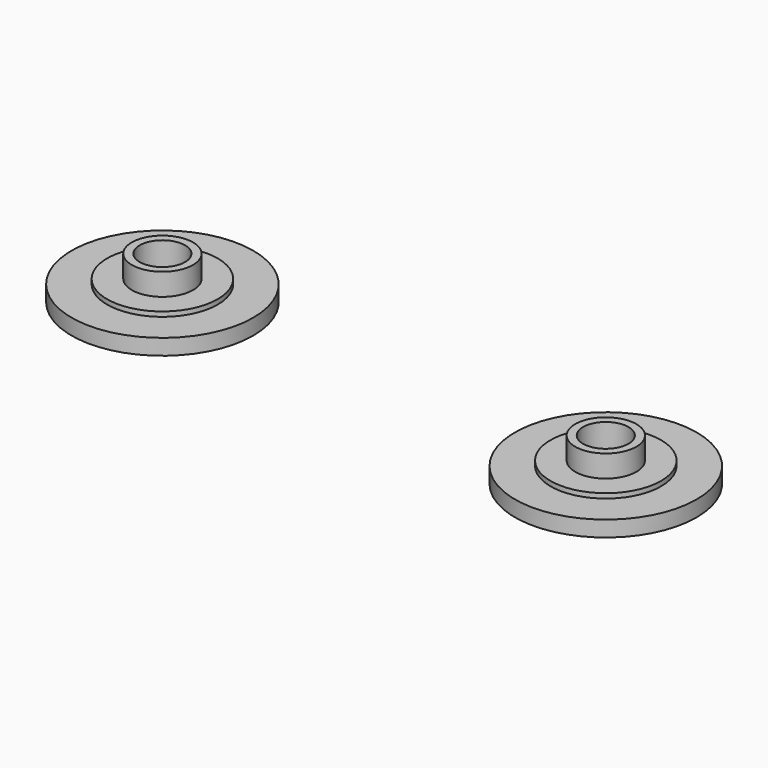
from build123d import *

# Parameters (mm, degrees)
F0_R        = 3.875
F1_DEPTH    = 3.4
F0_R_2      = 7
F2_DEPTH    = 0.6
F0_R_3      = 11.5
F3_DEPTH    = 2
F4_T        = 1
F5_R        = 3.875
F6_DEPTH    = 3.4
F5_R_2      = 7
F7_DEPTH    = 0.6
F6_FACE_R   = 3.875
F7_FACE_R   = 7
F7_FACE_R_2 = 3.875
F5_R_3      = 11.5
F8_DEPTH    = 2
F9_T        = 1


# Not quite as in the source:
# - a shell that OpenCascade refuses in one call is made with other operations: the cavity is built on its own and cut out


with BuildPart() as f1:
    # F0 (on Top) → F1 (new body)
    with BuildSketch(Plane.XY):
        Circle(F0_R)
    extrude(amount=F1_DEPTH)

    # F0 (on Top) → F2 (join)
    with BuildSketch(Plane.XY):
        Circle(F0_R_2)
        Circle(F0_R, mode=Mode.SUBTRACT)
    extrude(amount=F2_DEPTH)

    # F0 (on Top) → F3 (join)
    with BuildSketch(Plane.XY):
        Circle(F0_R_3)
        Circle(F0_R_2, mode=Mode.SUBTRACT)
        Circle(F0_R_2)
        Circle(F0_R, mode=Mode.SUBTRACT)
        Circle(F0_R)
    extrude(amount=-F3_DEPTH)

    # F4: shell of thickness 1, made by hand


with BuildPart() as f4_core1:
    # F4_t2: copy of F1
    add(f1.part)

    # the walls: a layer under each face that stays
    f4_faces = [f4_core1.faces().sort_by_distance(p)[0] for p in [
        (-11.5, 0, -1),
        (-7.6666666667, -7.6666666667, 0),
        (0, 0, -2),
        (-7, 0, 0.3),
        (-4.6666666667, -4.6666666667, 0.6),
        (-3.875, 0, 2),
    ]]
    thicken(f4_faces, amount=-F4_T, mode=Mode.SUBTRACT)

    # F4_s3 → F4_t4 (revolve, cut)
    with BuildSketch(Plane.XZ):
        Polygon((7.01, 0.01), (7, -1), (6, -1), (6, 0), align=None)
    revolve(axis=Axis((0, 0, 0), (0, 0, 1)), mode=Mode.SUBTRACT)

    # F4_s5 → F4_t6 (revolve, cut)
    with BuildSketch(Plane.XZ):
        Polygon((3.885, 0.61), (3.875, -0.4), (2.875, -0.4), (2.875, 0.6), align=None)
    revolve(axis=Axis((0, 0, 0.6), (0, 0, 1)), mode=Mode.SUBTRACT)


with BuildPart() as f1_1:
    add(f1.part)

    # what is left inside the walls is the cavity
    f4_cavity = [f4_core1.part.solids().sort_by_distance(p)[0] for p in [
        (0, -2, -0.99),
    ]]
    add(f4_cavity, mode=Mode.SUBTRACT)


with BuildPart() as f6:
    # F5 (on Top) → F6 (new body)
    with BuildSketch(Plane.XY):
        with Locations((-56.1332218349, 0)):
            Circle(F5_R)
    extrude(amount=F6_DEPTH)

    # F5 (on Top) → F7 (join)
    with BuildSketch(Plane.XY):
        with Locations((-56.1332218349, 0)):
            Circle(F5_R_2)
        with Locations((-56.1332218349, 0)):
            Circle(F5_R, mode=Mode.SUBTRACT)
    extrude(amount=F7_DEPTH)

    # F6_face (on face) + F7_face (on face) + F5 (on Top) → F8 (join)
    with BuildSketch(Plane(origin=(-56.1332218349, 0, 3.4), x_dir=(1, 0, 0), z_dir=(0, 0, 1))):
        Circle(F6_FACE_R)
    with BuildSketch(Plane(origin=(-56.1332218349, 0, 0.6), x_dir=(1, 0, 0), z_dir=(0, 0, 1))):
        Circle(F7_FACE_R)
        Circle(F7_FACE_R_2, mode=Mode.SUBTRACT)
    with BuildSketch(Plane.XY):
        with Locations((-56.1332218349, 0)):
            Circle(F5_R_3)
        with Locations((-56.1332218349, 0)):
            Circle(F5_R_2, mode=Mode.SUBTRACT)
    extrude(amount=F8_DEPTH)

    # F9: shell of thickness 1, made by hand


with BuildPart() as f9_core1:
    # F9_t2: copy of F6
    add(f6.part)

    # the walls: a layer under each face that stays
    f9_faces = [f9_core1.faces().sort_by_distance(p)[0] for p in [
        (-60.0082218349, 0, 4),
        (-60.7998885016, -4.6666666667, 2.6),
        (-63.1332218349, 0, 2.3),
        (-63.7998885016, -7.6666666667, 2),
        (-67.6332218349, 0, 1),
        (-56.1332218349, 0, 0),
    ]]
    thicken(f9_faces, amount=-F9_T, mode=Mode.SUBTRACT)

    # F9_s3 → F9_t4 (revolve, cut)
    with BuildSketch(Plane.XZ):
        Polygon((-52.2482218349, 2.61), (-53.2582218349, 2.6), (-53.2582218349, 1.6), (-52.2582218349, 1.6), align=None)
    revolve(axis=Axis((-56.1332218349, 0, 2.6), (0, 0, 1)), mode=Mode.SUBTRACT)

    # F9_s5 → F9_t6 (revolve, cut)
    with BuildSketch(Plane.XZ):
        Polygon((-49.1232218349, 2.01), (-50.1332218349, 2), (-50.1332218349, 1), (-49.1332218349, 1), align=None)
    revolve(axis=Axis((-56.1332218349, 0, 2), (0, 0, 1)), mode=Mode.SUBTRACT)


with BuildPart() as f6_1:
    add(f6.part)

    # what is left inside the walls is the cavity
    f9_cavity = [f9_core1.part.solids().sort_by_distance(p)[0] for p in [
        (-56.133222, -2, 1.01),
    ]]
    add(f9_cavity, mode=Mode.SUBTRACT)


solid = Compound([f1_1.part, f6_1.part])
